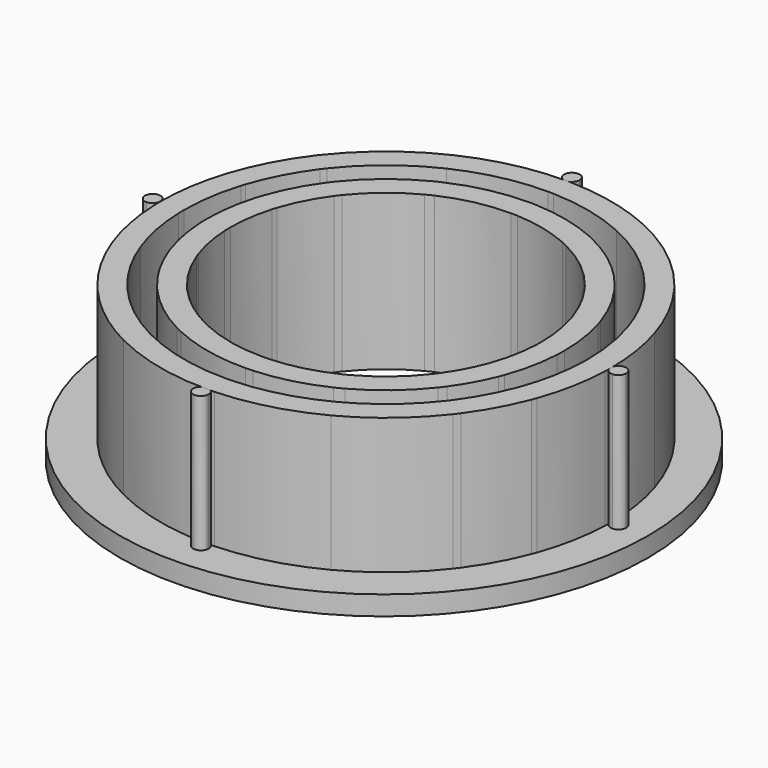
from build123d import *

# Parameters (mm, degrees)
F3_DEPTH = 25.4
F2_R     = 43.18
F2_R_2   = 25.4
F4_DEPTH = 3.175
F5_DEPTH = 25.4
F6_T     = -3.81


# Not quite as in the source:
# - a feature names something its author has since deleted; it is built from what else it names


with BuildPart() as f3:
    # F1 (on Top) → F3 (new body)
    with BuildSketch(Plane.XY):
        with BuildLine():
            ThreePointArc((-1.2683402303, 38.0788827706), (0, 38.1), (1.2683402303, 38.0788827706))
            ThreePointArc((1.2683402303, 38.0788827706), (0, 39.2839746803), (-1.2683402303, 38.0788827706))
        make_face()
        with BuildLine():
            ThreePointArc((-1.2683402303, 38.0788827706), (-0.032464654, 36.7443896905), (1.27, 38.0139746803))
            ThreePointArc((1.27, 38.0139746803), (1.2695849898, 38.0464393343), (1.2683402303, 38.0788827706))
            ThreePointArc((1.2683402303, 38.0788827706), (0, 38.1), (-1.2683402303, 38.0788827706))
        make_face()
    extrude(amount=F3_DEPTH)


with BuildPart() as f3b:
    # F1 (on Top) → F3, piece 2 (new body)
    with BuildSketch(Plane.XY):
        with BuildLine():
            ThreePointArc((-1.23848755, -38.0798653961), (0, -39.0687095881), (1.23848755, -38.0798653961))
            ThreePointArc((1.23848755, -38.0798653961), (0, -38.1), (-1.23848755, -38.0798653961))
        make_face()
        with BuildLine():
            ThreePointArc((-1.23848755, -38.0798653961), (0, -38.1), (1.23848755, -38.0798653961))
            ThreePointArc((1.23848755, -38.0798653961), (1.2620972998, -37.9401677293), (1.27, -37.7987095881))
            ThreePointArc((1.27, -37.7987095881), (-0.1414581413, -36.5366122882), (-1.23848755, -38.0798653961))
        make_face()
    extrude(amount=F3_DEPTH)


with BuildPart() as f3c:
    # F1 (on Top) → F3, piece 3 (new body)
    with BuildSketch(Plane.XY):
        with BuildLine():
            ThreePointArc((39.2839717627, 0), (38.934660903, 0.8747751178), (38.0788827756, 1.2683400807))
            ThreePointArc((38.0788827756, 1.2683400807), (38.0947203281, 0.6342579321), (38.1, 0))
            ThreePointArc((38.1, 0), (38.0947203281, -0.6342579321), (38.0788827756, -1.2683400807))
            ThreePointArc((38.0788827756, -1.2683400807), (38.934660903, -0.8747751178), (39.2839717627, 0))
        make_face()
        with BuildLine():
            ThreePointArc((38.1, 0), (38.0947203281, 0.6342579321), (38.0788827756, 1.2683400807))
            ThreePointArc((38.0788827756, 1.2683400807), (36.7439717627, 0), (38.0788827756, -1.2683400807))
            ThreePointArc((38.0788827756, -1.2683400807), (38.0947203281, -0.6342579321), (38.1, 0))
        make_face()
    extrude(amount=F3_DEPTH)


with BuildPart() as f3d:
    # F1 (on Top) → F3, piece 4 (new body)
    with BuildSketch(Plane.XY):
        with BuildLine():
            ThreePointArc((-38.0788514533, -1.2692801107), (-38.1, 0), (-38.0788514533, 1.2692801107))
            ThreePointArc((-38.0788514533, 1.2692801107), (-39.3916065753, 0), (-38.0788514533, -1.2692801107))
        make_face()
        with BuildLine():
            ThreePointArc((-36.8516065753, 0), (-37.2085898709, 0.8827799825), (-38.0788514533, 1.2692801107))
            ThreePointArc((-38.0788514533, 1.2692801107), (-38.1, 0), (-38.0788514533, -1.2692801107))
            ThreePointArc((-38.0788514533, -1.2692801107), (-37.2085898709, -0.8827799825), (-36.8516065753, 0))
        make_face()
    extrude(amount=F3_DEPTH)


with BuildPart() as f4:
    # F2 (on Top) → F4 (new body)
    with BuildSketch(Plane.XY):
        with Locations((-0.3331091177, 0.0348265304)):
            Circle(F2_R)
        with Locations((-0.3331091177, 0.0348265304)):
            Circle(F2_R_2, mode=Mode.SUBTRACT)
    extrude(amount=F4_DEPTH)


with BuildPart() as f5:
    # F0 (on Top) → F5 (new body)
    with BuildSketch(Plane.XY):
        with BuildLine():
            Line((36.83, 0), (25.4, 0))
            ThreePointArc((25.4, 0), (25.3920562906, -0.6351986588), (25.368230131, -1.2700000079))
            Line((25.368230131, -1.2700000079), (36.808096935, -1.2700000079))
            ThreePointArc((36.808096935, -1.2700000079), (36.8245238266, -0.6350944348), (36.83, 0))
        make_face()
        with BuildLine():
            ThreePointArc((24.3144775294, 7.3461678767), (25.12715393, 3.7129685397), (25.4, 0))
            Line((25.4, 0), (36.83, 0))
            ThreePointArc((36.83, 0), (36.405889268, 5.5731612761), (35.1433246479, 11.0179686284))
            Line((35.1433246479, 11.0179686284), (24.3144775294, 7.3461678767))
        make_face()
        with BuildLine():
            ThreePointArc((24.0831343406, 8.0723379719), (24.201529692, 7.7101206585), (24.3144775294, 7.3461678767))
            Line((24.3144775294, 7.3461678767), (35.1433246479, 11.0179686284))
            ThreePointArc((35.1433246479, 11.0179686284), (32.7990639639, 16.7532176938), (29.526562298, 22.0143366664))
            Line((29.526562298, 22.0143366664), (20.6123478246, 14.8422072873))
            ThreePointArc((20.6123478246, 14.8422072873), (22.602639539, 11.5879543436), (24.0831343406, 8.0723379719))
        make_face()
        with BuildLine():
            Line((36.808096935, -1.2700000079), (25.368230131, -1.2700000079))
            ThreePointArc((25.368230131, -1.2700000079), (24.8909275229, -5.0598149223), (23.8507080446, -8.7352003853))
            Line((23.8507080446, -8.7352003853), (34.6514763097, -12.4789458511))
            ThreePointArc((34.6514763097, -12.4789458511), (36.1666665427, -6.9585293841), (36.808096935, -1.2700000079))
        make_face()
        with BuildLine():
            Line((34.6514763097, -12.4789458511), (23.8507080446, -8.7352003853))
            ThreePointArc((23.8507080446, -8.7352003853), (23.7169249668, -9.0921653153), (23.5777996669, -9.447082241))
            Line((23.5777996669, -9.447082241), (34.3858203264, -13.1933415205))
            ThreePointArc((34.3858203264, -13.1933415205), (34.5204964043, -12.8368309173), (34.6514763097, -12.4789458511))
        make_face()
        with BuildLine():
            ThreePointArc((20.0019379644, 15.6551102733), (20.3112100908, 15.251712843), (20.6123478246, 14.8422072873))
            Line((20.6123478246, 14.8422072873), (29.526562298, 22.0143366664))
            ThreePointArc((29.526562298, 22.0143366664), (29.2200251868, 22.4196125765), (28.9079257527, 22.82062069))
            Line((28.9079257527, 22.82062069), (20.0019379644, 15.6551102733))
        make_face()
        with BuildLine():
            Line((34.3858203264, -13.1933415205), (23.5777996669, -9.447082241))
            ThreePointArc((23.5777996669, -9.447082241), (22.2466883618, -12.2574408802), (20.5821328328, -14.8840790126))
            Line((20.5821328328, -14.8840790126), (29.6846672935, -21.8006749363))
            ThreePointArc((29.6846672935, -21.8006749363), (32.3230319292, -17.6541923323), (34.3858203264, -13.1933415205))
        make_face()
        with BuildLine():
            ThreePointArc((11.1673735415, 22.8133681903), (15.9903614418, 19.7349522665), (20.0019379644, 15.6551102733))
            Line((20.0019379644, 15.6551102733), (28.9079257527, 22.82062069))
            ThreePointArc((28.9079257527, 22.82062069), (22.6834607768, 29.015676921), (15.1692978097, 33.5610086851))
            Line((15.1692978097, 33.5610086851), (10.2460415314, 23.2417433283))
            ThreePointArc((10.2460415314, 23.2417433283), (10.7088497321, 23.0321631076), (11.1673735415, 22.8133681903))
        make_face()
        with BuildLine():
            Line((29.6846672935, -21.8006749363), (20.5821328328, -14.8840790126))
            ThreePointArc((20.5821328328, -14.8840790126), (20.2803323476, -15.2927472963), (19.9704188085, -15.6952977867))
            Line((19.9704188085, -15.6952977867), (29.0720295756, -22.6111918384))
            ThreePointArc((29.0720295756, -22.6111918384), (29.3811434623, -22.2080460384), (29.6846672935, -21.8006749363))
        make_face()
        with BuildLine():
            Line((10.2460415314, 23.2417433283), (15.1692978097, 33.5610086851))
            ThreePointArc((15.1692978097, 33.5610086851), (8.3165271435, 35.8787440732), (1.1429013987, 36.8122625818))
            Line((1.1429013987, 36.8122625818), (1.1871979653, 25.3722399679))
            ThreePointArc((1.1871979653, 25.3722399679), (5.8150232442, 24.7254020123), (10.2460415314, 23.2417433283))
        make_face()
        with BuildLine():
            Line((29.0720295756, -22.6111918384), (19.9704188085, -15.6952977867))
            ThreePointArc((19.9704188085, -15.6952977867), (16.3560630102, -19.4329411775), (12.0563541506, -22.3563039118))
            Line((12.0563541506, -22.3563039118), (17.146194346, -32.5953511938))
            ThreePointArc((17.146194346, -32.5953511938), (23.6421639265, -28.239989109), (29.0720295756, -22.6111918384))
        make_face()
        with BuildLine():
            Line((1.1871979653, 25.3722399679), (1.1429013987, 36.8122625818))
            ThreePointArc((1.1429013987, 36.8122625818), (0.6349241086, 36.8245267638), (0.1268259647, 36.8297816335))
            Line((0.1268259647, 36.8297816335), (0.1710851086, 25.3994238101))
            ThreePointArc((0.1710851086, 25.3994238101), (0.6792775335, 25.3909153445), (1.1871979653, 25.3722399679))
        make_face()
        with BuildLine():
            Line((17.146194346, -32.5953511938), (12.0563541506, -22.3563039118))
            ThreePointArc((12.0563541506, -22.3563039118), (11.4936590793, -22.6507351088), (10.9237788592, -22.93100642))
            ThreePointArc((10.9237788592, -22.93100642), (6.2726353013, -24.6132900356), (1.3836455916, -25.3622854821))
            Line((1.3836455916, -25.3622854821), (1.4279421582, -36.802308096))
            ThreePointArc((1.4279421582, -36.802308096), (9.5223032042, -35.5777267639), (17.146194346, -32.5953511938))
        make_face()
        with BuildLine():
            Line((0.1710851086, 25.3994238101), (0.1268259647, 36.8297816335))
            ThreePointArc((0.1268259647, 36.8297816335), (-7.9466571571, 35.9624740532), (-15.633874534, 33.3471268186))
            Line((-15.633874534, 33.3471268186), (-10.5440343386, 23.1080795365))
            ThreePointArc((-10.5440343386, 23.1080795365), (-5.3115048317, 24.8384362717), (0.1710851086, 25.3994238101))
        make_face()
        with BuildLine():
            Line((-10.5440343386, 23.1080795365), (-15.633874534, 33.3471268186))
            ThreePointArc((-15.633874534, 33.3471268186), (-22.915404324, 28.8328483621), (-28.9569488784, 22.7583833269))
            Line((-28.9569488784, 22.7583833269), (-19.8544144177, 15.8417874032))
            ThreePointArc((-19.8544144177, 15.8417874032), (-16.1231392327, 19.6266242967), (-11.6859355325, 22.5521376089))
            ThreePointArc((-11.6859355325, 22.5521376089), (-11.1184602339, 22.8372468136), (-10.5440343386, 23.1080795365))
        make_face()
        with BuildLine():
            Line((1.4279421582, -36.802308096), (1.3836455916, -25.3622854821))
            ThreePointArc((1.3836455916, -25.3622854821), (0.8758850125, -25.3848936465), (0.3677737157, -25.3973373111))
            Line((0.3677737157, -25.3973373111), (0.4120328596, -36.8276951345))
            ThreePointArc((0.4120328596, -36.8276951345), (0.9200750741, -36.8185056983), (1.4279421582, -36.802308096))
        make_face()
        with BuildLine():
            Line((-19.8544144177, 15.8417874032), (-28.9569488784, 22.7583833269))
            ThreePointArc((-28.9569488784, 22.7583833269), (-29.2681039466, 22.3568108497), (-29.5736904662, 21.9509847663))
            Line((-29.5736904662, 21.9509847663), (-20.472079699, 15.0350907146))
            ThreePointArc((-20.472079699, 15.0350907146), (-20.1672809725, 15.4415277151), (-19.8544144177, 15.8417874032))
        make_face()
        with BuildLine():
            Line((0.4120328596, -36.8276951345), (0.3677737157, -25.3973373111))
            ThreePointArc((0.3677737157, -25.3973373111), (-5.3024594537, -24.8403688327), (-10.7058949976, -23.0335366868))
            ThreePointArc((-10.7058949976, -23.0335366868), (-11.164446871, -22.8148005923), (-11.6185320778, -22.5869367635))
            Line((-11.6185320778, -22.5869367635), (-16.5417883561, -32.9062021203))
            ThreePointArc((-16.5417883561, -32.9062021203), (-8.2998060194, -35.8826158472), (0.4120328596, -36.8276951345))
        make_face()
        with BuildLine():
            Line((-20.472079699, 15.0350907146), (-29.5736904662, 21.9509847663))
            ThreePointArc((-29.5736904662, 21.9509847663), (-32.6665719132, 17.0101140337), (-34.941178027, 11.643151553))
            Line((-34.941178027, 11.643151553), (-24.1404097619, 7.8994060871))
            ThreePointArc((-24.1404097619, 7.8994060871), (-22.5897776162, 11.6130076746), (-20.472079699, 15.0350907146))
        make_face()
        with BuildLine():
            ThreePointArc((-27.8250317592, -24.1291630108), (-22.6133320337, -29.0703648813), (-16.5417883561, -32.9062021203))
            Line((-16.5417883561, -32.9062021203), (-11.6185320778, -22.5869367635))
            ThreePointArc((-11.6185320778, -22.5869367635), (-15.5220567406, -20.105366312), (-18.9108172857, -16.9570336317))
            Line((-18.9108172857, -16.9570336317), (-27.8250317592, -24.1291630108))
        make_face()
        with BuildLine():
            Line((-24.1404097619, 7.8994060871), (-34.941178027, 11.643151553))
            ThreePointArc((-34.941178027, 11.643151553), (-35.0597839174, 11.2809774251), (-35.1746358928, 10.9175954223))
            Line((-35.1746358928, 10.9175954223), (-24.3666152333, 7.1713361428))
            ThreePointArc((-24.3666152333, 7.1713361428), (-24.2562443493, 7.5362198793), (-24.1404097619, 7.8994060871))
        make_face()
        with BuildLine():
            ThreePointArc((-28.4801844464, -23.3522588607), (-28.1552879226, -23.7429707913), (-27.8250317592, -24.1291630108))
            Line((-27.8250317592, -24.1291630108), (-18.9108172857, -16.9570336317))
            ThreePointArc((-18.9108172857, -16.9570336317), (-19.2463609387, -16.5752101229), (-19.5741966581, -16.186748444))
            Line((-19.5741966581, -16.186748444), (-28.4801844464, -23.3522588607))
        make_face()
        with BuildLine():
            Line((-24.3666152333, 7.1713361428), (-35.1746358928, 10.9175954223))
            ThreePointArc((-35.1746358928, 10.9175954223), (-36.4138074083, 5.5211891865), (-36.83, 0))
            Line((-36.83, 0), (-25.4, 0))
            ThreePointArc((-25.4, 0), (-25.1403264391, 3.6227043127), (-24.3666152333, 7.1713361428))
        make_face()
        with BuildLine():
            ThreePointArc((-34.5969673319, -12.6292815091), (-31.9910507789, -18.2488785974), (-28.4801844464, -23.3522588607))
            Line((-28.4801844464, -23.3522588607), (-19.5741966581, -16.186748444))
            ThreePointArc((-19.5741966581, -16.186748444), (-21.9705413172, -12.7457959434), (-23.7681202134, -8.9574807574))
            Line((-23.7681202134, -8.9574807574), (-34.5969673319, -12.6292815091))
        make_face()
        with BuildLine():
            Line((-25.4, 0), (-36.83, 0))
            ThreePointArc((-36.83, 0), (-36.8245238266, -0.6350944348), (-36.808096935, -1.2700000079))
            Line((-36.808096935, -1.2700000079), (-25.368230131, -1.2700000079))
            ThreePointArc((-25.368230131, -1.2700000079), (-25.3920562906, -0.6351986588), (-25.4, 0))
        make_face()
        with BuildLine():
            ThreePointArc((-36.808096935, -1.2700000079), (-36.1514746559, -7.0370292171), (-34.5969673319, -12.6292815091))
            Line((-34.5969673319, -12.6292815091), (-23.7681202134, -8.9574807574))
            ThreePointArc((-23.7681202134, -8.9574807574), (-23.8998304311, -8.5998898461), (-24.0261610442, -8.2403631884))
            ThreePointArc((-24.0261610442, -8.2403631884), (-24.9418916807, -4.8022952211), (-25.368230131, -1.2700000079))
            Line((-25.368230131, -1.2700000079), (-36.808096935, -1.2700000079))
        make_face()
    extrude(amount=F5_DEPTH)

    # F6
    f6_openings = [f5.faces().sort_by_distance(p)[0] for p in [
        (24.742903, 9.324847, 25.4),
    ]]
    offset(amount=F6_T, openings=f6_openings)


solid = Compound([f3.part, f3b.part, f3c.part, f3d.part, f4.part, f5.part])
